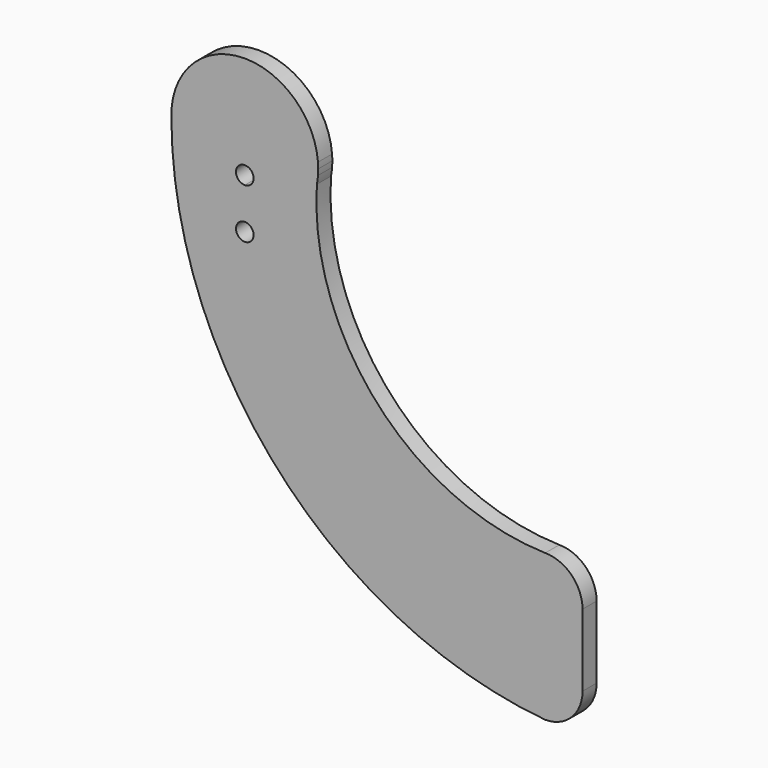
from build123d import *

# Parameters (mm, degrees)
F0_R     = 1.5
F1_DEPTH = 3
F3_DEPTH = 381


with BuildPart() as f1:
    # F0 (on Front) → F1 (new body)
    with BuildSketch(Plane.XZ):
        with BuildLine():
            ThreePointArc((12.4599357944, -0.3280291537), (12.4796291372, -0.163973202), (12.5, 0))
            ThreePointArc((12.5, 0), (12.4899799325, 0.5004011242), (12.4599357944, 1))
            Line((12.4599357944, 1), (12.4599357944, -0.3280291537))
        make_face()
        with BuildLine():
            ThreePointArc((12.4599357944, -1), (12.4899799325, -0.5004011242), (12.5, 0))
            ThreePointArc((12.5, 0), (12.4796291372, -0.163973202), (12.4599357944, -0.3280291537))
            Line((12.4599357944, -0.3280291537), (12.4599357944, -1))
        make_face()
        with BuildLine():
            Line((12.4599357944, -0.3280291537), (12.4599357944, 1))
            ThreePointArc((12.4599357944, 1), (0, 12.5), (-12.4599357944, 1))
            Line((-12.4599357944, 1), (-12.4599357944, -1))
            ThreePointArc((-12.4599357944, -1), (-0.696307501, -12.4805911664), (12.2713731569, -2.3797900839))
            ThreePointArc((12.2713731569, -2.3797900839), (12.3524414608, -1.3526953053), (12.4599357944, -0.3280291537))
        make_face()
        Circle(F0_R, mode=Mode.SUBTRACT)
        with BuildLine():
            ThreePointArc((12.2713731569, -2.3797900839), (12.3848845687, -1.6925230338), (12.4599357944, -1))
            Line((12.4599357944, -1), (12.4599357944, -0.3280291537))
            ThreePointArc((12.4599357944, -0.3280291537), (12.3524414608, -1.3526953053), (12.2713731569, -2.3797900839))
        make_face()
        with BuildLine():
            Line((-12.4599357944, -1), (-12.4599357944, 1))
            ThreePointArc((-12.4599357944, 1), (-12.4899799325, 0.5004011242), (-12.5, 0))
            ThreePointArc((-12.5, 0), (-12.4899799325, -0.5004011242), (-12.4599357944, -1))
        make_face()
        with BuildLine():
            ThreePointArc((51.15, -45), (22.6329157643, -31.9707379741), (12.2713731569, -2.3797900839))
            ThreePointArc((12.2713731569, -2.3797900839), (-0.696307501, -12.4805911664), (-12.4599357944, -1))
            ThreePointArc((-12.4599357944, -1), (-12.4899799325, -0.5004011242), (-12.5, 0))
            Line((-12.5, 0), (-12.5, -0.5771173286))
            ThreePointArc((-12.5, -0.5771173286), (5.9031905044, -47.5942731711), (51.15, -70))
            ThreePointArc((51.15, -70), (55.6401280605, -68.1401280605), (57.5, -63.65))
            Line((57.5, -63.65), (57.5, -51.35))
            ThreePointArc((57.5, -51.35), (55.6401280605, -46.8598719395), (51.15, -45))
        make_face()
        with BuildLine():
            Line((-12.5, -0.5771173286), (-12.5, 0))
            ThreePointArc((-12.5, 0), (-12.5005947604, -0.2885586643), (-12.5, -0.5771173286))
        make_face()
        Circle(F0_R)
    extrude(amount=F1_DEPTH)

    # F2 (on face) → F3 (cut, symmetric)
    with BuildSketch(Plane.XZ.offset(3)):
        with BuildLine():
            ThreePointArc((1.5, -5), (1.0606601718, -3.9393398282), (0, -3.5))
            Line((0, -3.5), (0, -5))
            Line((0, -5), (0, -6.5))
            ThreePointArc((0, -6.5), (1.0606601718, -6.0606601718), (1.5, -5))
        make_face()
        with BuildLine():
            ThreePointArc((1.5, -13.5), (1.0606601718, -12.4393398282), (0, -12))
            ThreePointArc((0, -12), (-1.0606601718, -14.5606601718), (1.5, -13.5))
        make_face()
        with BuildLine():
            Line((0, -5), (0, -3.5))
            ThreePointArc((0, -3.5), (-1.5, -5), (0, -6.5))
            Line((0, -6.5), (0, -5))
        make_face()
    extrude(amount=F3_DEPTH, both=True, mode=Mode.SUBTRACT)


solid = f1.part
